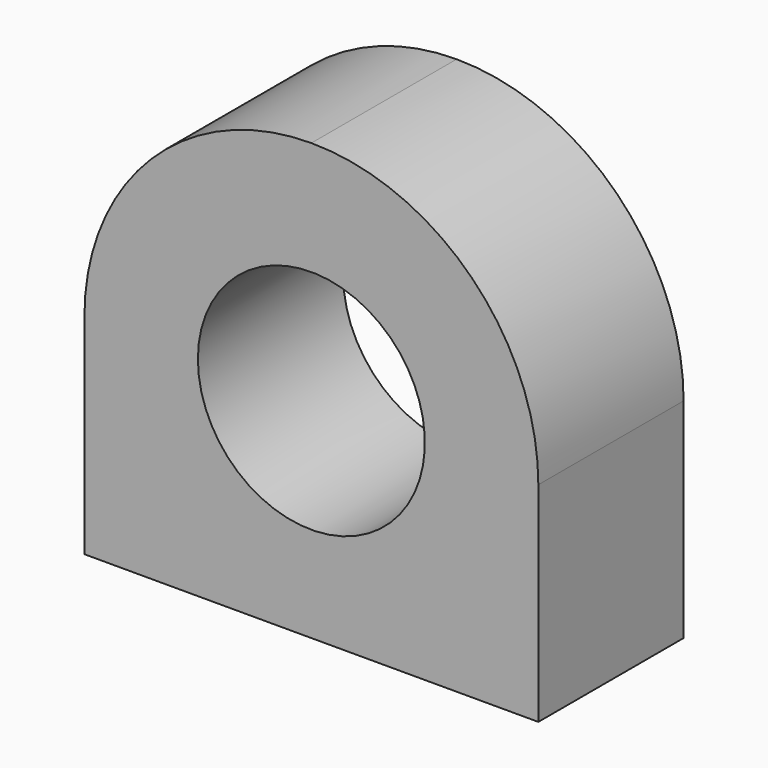
from build123d import *

# Parameters (mm, degrees)
F0_W     = 50
F0_H     = 48
F1_DEPTH = 20
F2_R     = 24.99999
F3_R     = 12.5
F4_DEPTH = 25


# Not quite as in the source:
# - a fillet or chamfer is up to 0.001 mm smaller than in the source, because OpenCascade refuses the exact size


with BuildPart() as f1:
    # F0 (on Front) → F1 (new body)
    with BuildSketch(Plane.XZ):
        with Locations((-20.5971896648, 6.0340394775)):
            Rectangle(F0_W, F0_H)
    extrude(amount=F1_DEPTH)

    # F2 (radius 25 in the source; OpenCascade refuses exactly that, so slightly less here)
    f2_edges = [f1.edges().sort_by_distance(p)[0] for p in [
        (4.40281, -10, 30.034039),
        (-45.59719, -10, 30.034039),
    ]]
    fillet(f2_edges, radius=F2_R)

    # F3 (on face) → F4 (cut)
    with BuildSketch(Plane(origin=(0, 0, 0), x_dir=(-1, 0, 0), z_dir=(0, 1, 0))):
        with Locations((20.5971896648, 5.0340394775)):
            Circle(F3_R)
    extrude(amount=-F4_DEPTH, mode=Mode.SUBTRACT)


solid = f1.part
